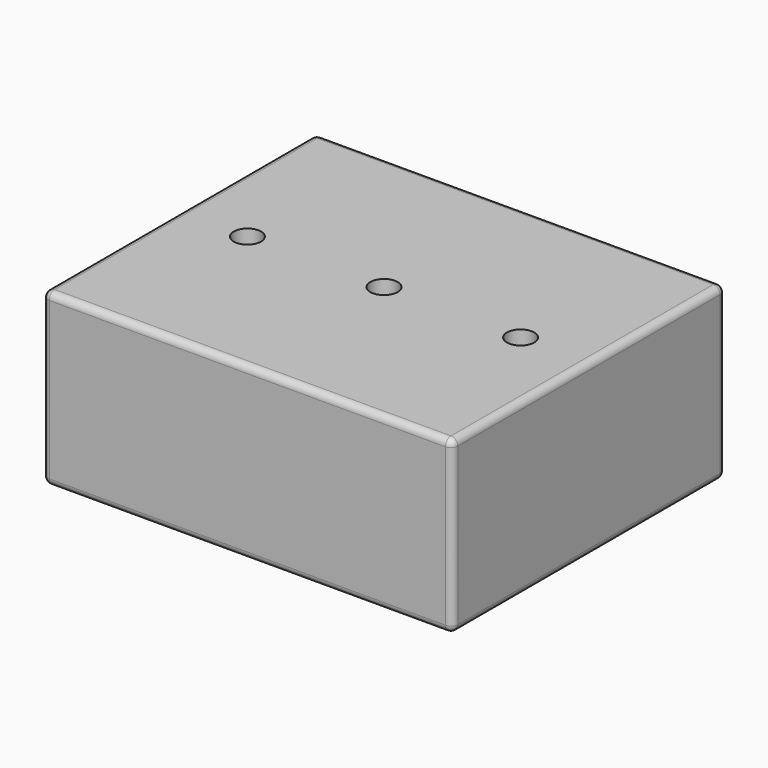
from build123d import *

# Parameters (mm, degrees)
F0_W     = 30.48
F0_H     = 25.4
F0_R     = 1.016
F1_DEPTH = 12.7
F2_R     = 0.508


# Not quite as in the source:
# - a feature names something its author has since deleted; it is built from what else it names


with BuildPart() as f1:
    # F0 (on Top) → F1 (new body)
    with BuildSketch(Plane.XY):
        with Locations((-46.7100512166, 5.7338142046)):
            Rectangle(F0_W, F0_H)
        with Locations((-56.8700512166, 5.7338142046)):
            Circle(F0_R, mode=Mode.SUBTRACT)
        with Locations((-46.7100512166, 5.7338142046)):
            Circle(F0_R, mode=Mode.SUBTRACT)
        with Locations((-36.5500512166, 5.7338142046)):
            Circle(F0_R, mode=Mode.SUBTRACT)
    extrude(amount=-F1_DEPTH)

    # F2
    f2_edges = [f1.edges().sort_by_distance(p)[0] for p in [
        (-46.710051, 18.433814, 0),
        (-61.950051, 5.733814, 0),
        (-61.950051, 18.433814, -6.35),
        (-46.710051, 18.433814, -12.7),
        (-61.950051, 5.733814, -12.7),
        (-31.470051, 5.733814, 0),
        (-46.710051, -6.966186, 0),
        (-31.470051, -6.966186, -6.35),
        (-31.470051, 5.733814, -12.7),
        (-46.710051, -6.966186, -12.7),
        (-31.470051, 18.433814, -6.35),
        (-61.950051, -6.966186, -6.35),
    ]]
    fillet(f2_edges, radius=F2_R)


solid = f1.part
